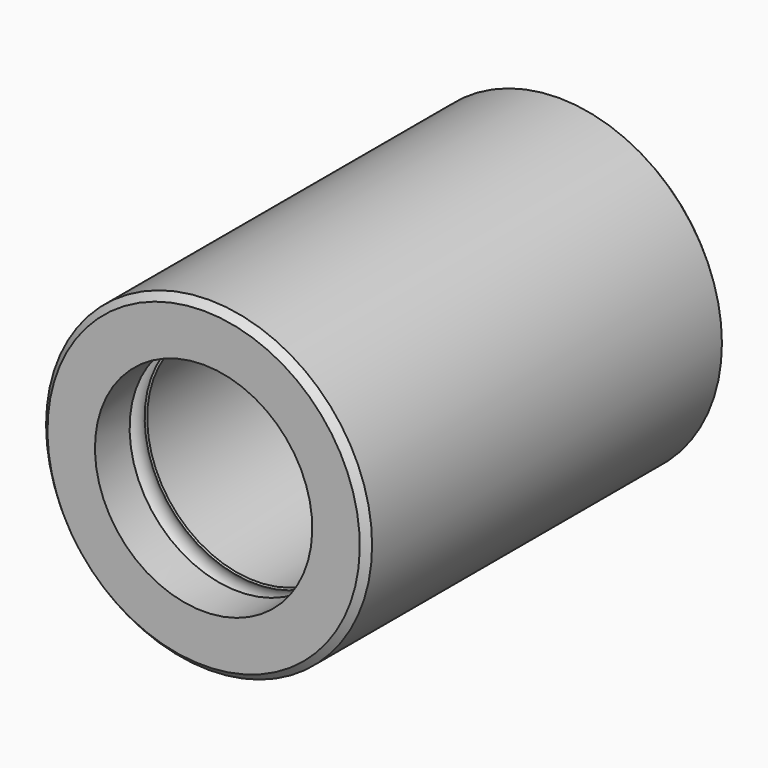
from build123d import *

# Parameters (mm, degrees)
F3_SIZE = 1.6002


# Not quite as in the source:
# - a fillet or chamfer that OpenCascade refuses, or shapes differently, is made with other operations: its cross-section is extruded or revolved along the edge and cut away or added


with BuildPart() as f1:
    # F0 (on Right) → F1 (revolve)
    with BuildSketch(Plane.YZ):
        with BuildLine():
            Line((105.41, 38.1), (0, 38.1))
            Line((0, 38.1), (0, 25.4))
            Line((0, 25.4), (10.795, 25.4))
            ThreePointArc((10.795, 25.4), (12.7, 31.115), (14.605, 25.4))
            Line((14.605, 25.4), (90.805, 25.4))
            ThreePointArc((90.805, 25.4), (92.71, 31.115), (94.615, 25.4))
            Line((94.615, 25.4), (105.41, 25.4))
            Line((105.41, 25.4), (105.41, 38.1))
        make_face()
    revolve(axis=Axis((0, 63.5, 0), (0, 1, 0)))

    # F2: chamfer of 0.7874 on 6 edges, made by hand

    # F2_s1 → F2_t2 (revolve, cut)
    with BuildSketch(Plane.YZ):
        with BuildLine():
            Line((10.1123747416, 25.3712836476), (10.3348384737, 25.8650833474))
            Line((10.3348384737, 25.8650833474), (10.346633843, 25.8755173671))
            ThreePointArc((10.346633843, 25.8755173671), (10.5543660431, 25.6211364589), (10.8044488, 25.4125984))
            Line((10.8044488, 25.4125984), (10.795, 25.384252))
            ThreePointArc((10.795, 25.384252), (10.4536873708, 25.384252), (10.1123747416, 25.3555356476))
            Line((10.1123747416, 25.3555356476), (10.1123747416, 25.3712836476))
        make_face()
    revolve(axis=Axis((0, 10.795, 0), (0, 1, 0)), mode=Mode.SUBTRACT)

    # F2_s3 → F2_t4 (revolve, cut)
    with BuildSketch(Plane.YZ):
        with BuildLine():
            Line((15.0651615263, 25.8650833474), (15.2876252584, 25.3712836476))
            Line((15.2876252584, 25.3712836476), (15.2876252584, 25.3555356476))
            ThreePointArc((15.2876252584, 25.3555356476), (14.9463126292, 25.384252), (14.605, 25.384252))
            Line((14.605, 25.384252), (14.5955512, 25.4125984))
            ThreePointArc((14.5955512, 25.4125984), (14.8456339569, 25.6211364589), (15.053366157, 25.8755173671))
            Line((15.053366157, 25.8755173671), (15.0651615263, 25.8650833474))
        make_face()
    revolve(axis=Axis((0, 14.605, 0), (0, 1, 0)), mode=Mode.SUBTRACT)

    # F2_s5 → F2_t6 (revolve, cut)
    with BuildSketch(Plane.YZ):
        with BuildLine():
            Line((90.1223747416, 25.3712836476), (90.3448384737, 25.8650833474))
            Line((90.3448384737, 25.8650833474), (90.356633843, 25.8755173671))
            ThreePointArc((90.356633843, 25.8755173671), (90.5643660431, 25.6211364589), (90.8144488, 25.4125984))
            Line((90.8144488, 25.4125984), (90.805, 25.384252))
            ThreePointArc((90.805, 25.384252), (90.4636873708, 25.384252), (90.1223747416, 25.3555356476))
            Line((90.1223747416, 25.3555356476), (90.1223747416, 25.3712836476))
        make_face()
    revolve(axis=Axis((0, 90.805, 0), (0, 1, 0)), mode=Mode.SUBTRACT)

    # F2_s7 → F2_t8 (revolve, cut)
    with BuildSketch(Plane.YZ):
        with BuildLine():
            Line((95.2976252584, 25.3712836476), (95.0751615263, 25.8650833474))
            Line((95.0751615263, 25.8650833474), (95.063366157, 25.8755173671))
            ThreePointArc((95.063366157, 25.8755173671), (94.8556339569, 25.6211364589), (94.6055512, 25.4125984))
            Line((94.6055512, 25.4125984), (94.615, 25.384252))
            ThreePointArc((94.615, 25.384252), (94.9563126292, 25.384252), (95.2976252584, 25.3555356476))
            Line((95.2976252584, 25.3555356476), (95.2976252584, 25.3712836476))
        make_face()
    revolve(axis=Axis((0, 94.615, 0), (0, 1, 0)), mode=Mode.SUBTRACT)

    # F3
    f3_edges = [f1.edges().sort_by_distance(p)[0] for p in [
        (0, 105.41, -38.1),
        (0, 0, -38.1),
    ]]
    chamfer(f3_edges, length=F3_SIZE)


solid = f1.part
